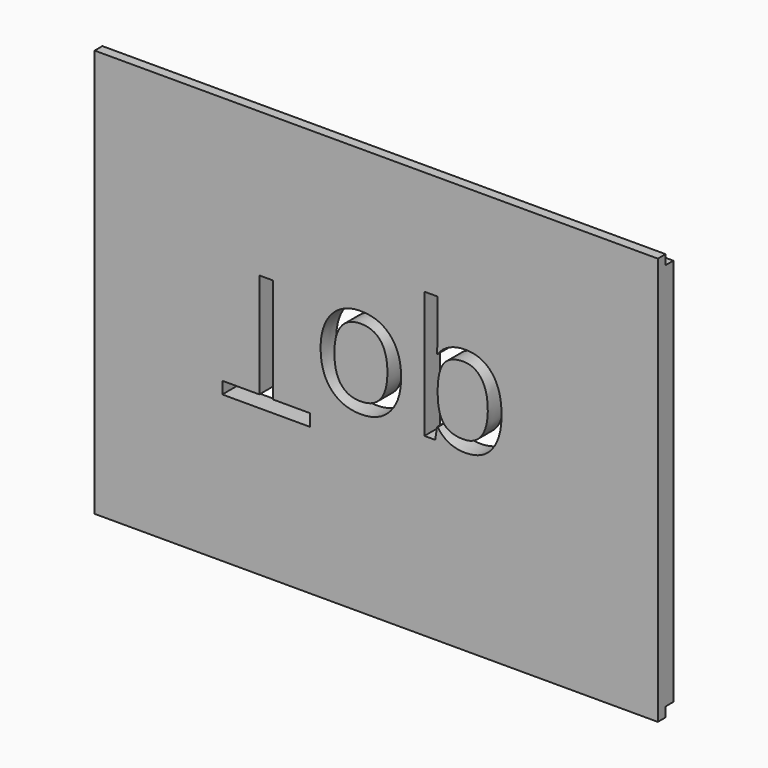
from build123d import *

# Parameters (mm, degrees)
F0_W         = 145
F0_H         = 100
F1_DEPTH     = 5
F2_TEXT_SIZE = 42.1496311907
F3_DEPTH     = 5
F4_W         = 145
F4_H         = 2.5
F5_DEPTH     = 2.5
F7_DEPTH     = 2.5
F6_W         = 145
F6_H         = 2.5
F8_DEPTH     = 2.5


# Not quite as in the source:
# - Text() gives the source's letters only with a copy of the font that has no kerning and outlines rounded to 1/6400 em; it was checked with that copy


with BuildPart() as f1:
    # F0 (on Front) → F1 (new body)
    with BuildSketch(Plane.XZ):
        with Locations((2.5, -2.5)):
            Rectangle(F0_W, F0_H)
    extrude(amount=F1_DEPTH)

    # F2 (on face) → F3 (cut)
    with BuildSketch(Plane(origin=(0, 0, 0), x_dir=(-1, 0, 0), z_dir=(0, 1, 0))):
        with Locations(Location((37.5, 12.8387018896), (0, 0, -180))):
            Text('Top', F2_TEXT_SIZE, font='Open Sans', text_align=(TextAlign.LEFT, TextAlign.BOTTOM))
    extrude(amount=-F3_DEPTH, mode=Mode.SUBTRACT)

    # F4 (on face) → F5 (join)
    with BuildSketch(Plane(origin=(0, 0, -52.5), x_dir=(1, 0, 0), z_dir=(0, 0, -1))):
        with Locations((2.5, 3.75)):
            Rectangle(F4_W, F4_H)
    extrude(amount=F5_DEPTH)

    # F4 (on face) → F7 (join)
    with BuildSketch(Plane(origin=(0, 0, -52.5), x_dir=(1, 0, 0), z_dir=(0, 0, -1))):
        with Locations((2.5, 3.75)):
            Rectangle(F4_W, F4_H)
    extrude(amount=F7_DEPTH)

    # F6 (on face) → F8 (join)
    with BuildSketch(Plane.XY.offset(47.5)):
        with Locations((2.5, -3.75)):
            Rectangle(F6_W, F6_H)
    extrude(amount=F8_DEPTH)


solid = f1.part
